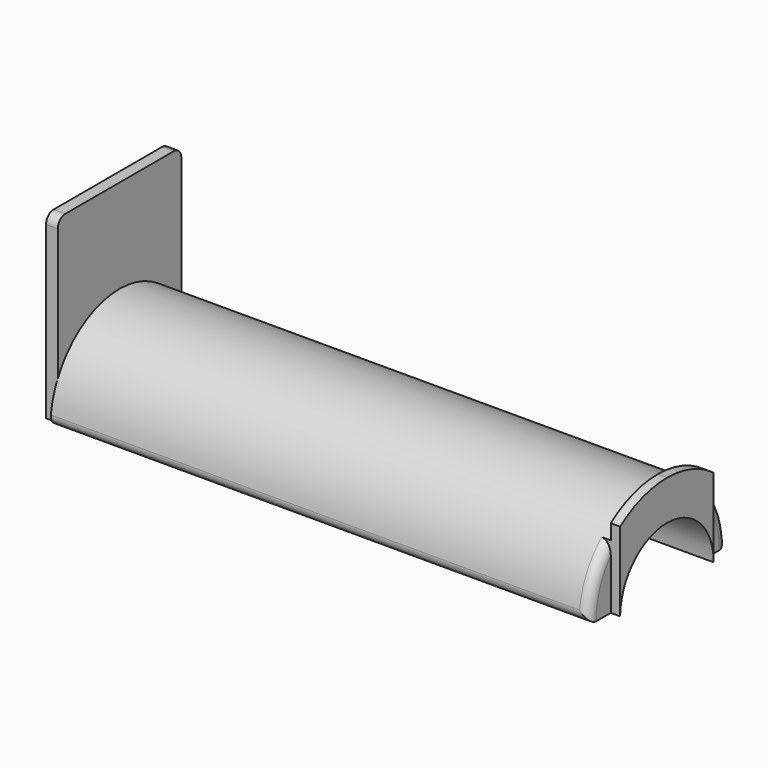
from build123d import *

# Parameters (mm, degrees)
F1_DEPTH     = 115
F3_DEPTH     = 2
F5_DEPTH     = 2.5
F6_R         = 2
F8_DEPTH     = 5
F10_DEPTH    = 119.5
F11_T1_DEPTH = 126.2328463215
F11_T6_ANGLE = 78.4675131369
F12_T1_DEPTH = 124.2328463215
F12_T6_ANGLE = 71.5045093033


# Not quite as in the source:
# - a fillet or chamfer that OpenCascade refuses, or shapes differently, is made with other operations: its cross-section is extruded or revolved along the edge and cut away or added


with BuildPart() as f1:
    # F0 (on Right) → F1 (new body)
    with BuildSketch(Plane.YZ):
        with BuildLine():
            Line((-18.5, 0), (18.5, 0))
            ThreePointArc((18.5, 0), (0, 18.5), (-18.5, 0))
        make_face()
    extrude(amount=-F1_DEPTH)

    # F2 (on face) → F3 (join)
    with BuildSketch(Plane.YZ):
        with BuildLine():
            Line((12.5, 21), (-12.5, 21))
            Line((-12.5, 21), (-12.5, 13.638181697))
            ThreePointArc((-12.5, 13.638181697), (0, 18.5), (12.5, 13.638181697))
            Line((12.5, 13.638181697), (12.5, 21))
        make_face()
        with BuildLine():
            ThreePointArc((12.5, 13.638181697), (0, 18.5), (-12.5, 13.638181697))
            Line((-12.5, 13.638181697), (-12.5, 0))
            Line((-12.5, 0), (12.5, 0))
            Line((12.5, 0), (12.5, 13.638181697))
        make_face()
    extrude(amount=F3_DEPTH)

    # F4 (on face) → F5 (join)
    with BuildSketch(Plane(origin=(-115, 0, 0), x_dir=(0, -1, 0), z_dir=(-1, 0, 0))):
        with BuildLine():
            Line((-16.5, 8.3666002653), (-16.5, 0))
            Line((-16.5, 0), (16.5, 0))
            Line((16.5, 0), (16.5, 8.3666002653))
            ThreePointArc((16.5, 8.3666002653), (0, 18.5), (-16.5, 8.3666002653))
        make_face()
        with BuildLine():
            Line((-16.5, 38.5), (-16.5, 8.3666002653))
            ThreePointArc((-16.5, 8.3666002653), (0, 18.5), (16.5, 8.3666002653))
            Line((16.5, 8.3666002653), (16.5, 38.5))
            Line((16.5, 38.5), (-16.5, 38.5))
        make_face()
    extrude(amount=F5_DEPTH)

    # F6
    f6_edges = [f1.edges().sort_by_distance(p)[0] for p in [
        (-116.25, 16.5, 38.5),
        (-116.25, -16.5, 38.5),
    ]]
    fillet(f6_edges, radius=F6_R)

    # F7 (on face) → F8 (cut)
    with BuildSketch(Plane.YZ.offset(2)):
        with BuildLine():
            Line((-12.5, 21), (-12.5, 16.8745370307))
            ThreePointArc((-12.5, 16.8745370307), (-6.5815925928, 19.9419818208), (1.93e-08, 21))
            Line((1.93e-08, 21), (-12.5, 21))
        make_face()
        with BuildLine():
            ThreePointArc((1.93e-08, 21), (6.5815926111, 19.9419818148), (12.5, 16.8745370307))
            Line((12.5, 16.8745370307), (12.5, 21))
            Line((12.5, 21), (1.93e-08, 21))
        make_face()
    extrude(amount=-F8_DEPTH, mode=Mode.SUBTRACT)

    # F9 (on face) → F10 (cut, through all)
    with BuildSketch(Plane.YZ.offset(2)):
        with BuildLine():
            Line((-12.5, 0), (12.5, 0))
            ThreePointArc((12.5, 0), (0, 12.5), (-12.5, 0))
        make_face()
    extrude(amount=-F10_DEPTH, mode=Mode.SUBTRACT)

    # F11: fillet of radius 2 on 2 edges, made by hand

    # F11_s2 → F11_t1 (cut)
    with BuildSketch(Plane.YZ.offset(-120.6164231607)):
        with BuildLine():
            ThreePointArc((18.3635926092, 2.2424242424), (17.8758119724, 0.6742640694), (16.3783393542, 0))
            Line((16.3783393542, 0), (18.5, 0))
            ThreePointArc((18.5, 0), (18.4658666635, 1.1232846321), (18.3635926092, 2.2424242424))
        make_face()
    extrude(amount=F11_T1_DEPTH, mode=Mode.SUBTRACT)


with BuildPart() as f11_tool4:
    # F11_s5 → F11_t6 (revolve)
    with BuildSketch(Plane(origin=(0, 0, 0), x_dir=(1, 0, 0), z_dir=(0, 0.8908514497, 0.454294722))):
        with BuildLine():
            ThreePointArc((-2, -18.5), (-0.5857864376, -17.9142135624), (0, -16.5))
            Line((0, -16.5), (0, -18.5))
            Line((0, -18.5), (-2, -18.5))
        make_face()
    revolve(axis=Axis((0, 0, 0), (1, 0, 0)), revolution_arc=F11_T6_ANGLE)

    split(bisect_by=Plane.XZ.offset(12.5), keep=Keep.TOP)


with BuildPart() as f1_1:
    add(f1.part)

    # F11_t3: cut F11_tool4
    add(f11_tool4.part, mode=Mode.SUBTRACT)

    # F12: fillet of radius 2 on 2 edges, made by hand

    # F12_s2 → F12_t1 (cut)
    with BuildSketch(Plane.YZ.offset(-120.6164231607)):
        with BuildLine():
            ThreePointArc((-18.3635926092, 2.2424242424), (-17.8758119724, 0.6742640694), (-16.3783393542, 0))
            Line((-16.3783393542, 0), (-18.5, 0))
            ThreePointArc((-18.5, 0), (-18.4658666635, 1.1232846321), (-18.3635926092, 2.2424242424))
        make_face()
    extrude(amount=F12_T1_DEPTH, mode=Mode.SUBTRACT)


with BuildPart() as f12_tool4:
    # F12_s5 → F12_t6 (revolve)
    with BuildSketch(Plane(origin=(0, 0, 0), x_dir=(1, 0, 0), z_dir=(0, -0.1482330737, -0.9889524538))):
        with BuildLine():
            ThreePointArc((-2, -18.5), (-0.5857864376, -17.9142135624), (0, -16.5))
            Line((0, -16.5), (0, -18.5))
            Line((0, -18.5), (-2, -18.5))
        make_face()
    revolve(axis=Axis((0, 0, 0), (1, 0, 0)), revolution_arc=F12_T6_ANGLE)

    split(bisect_by=Plane.XZ.offset(-12.5), keep=Keep.BOTTOM)


with BuildPart() as f1_2:
    add(f1_1.part)

    # F12_t3: cut F12_tool4
    add(f12_tool4.part, mode=Mode.SUBTRACT)


solid = f1_2.part
